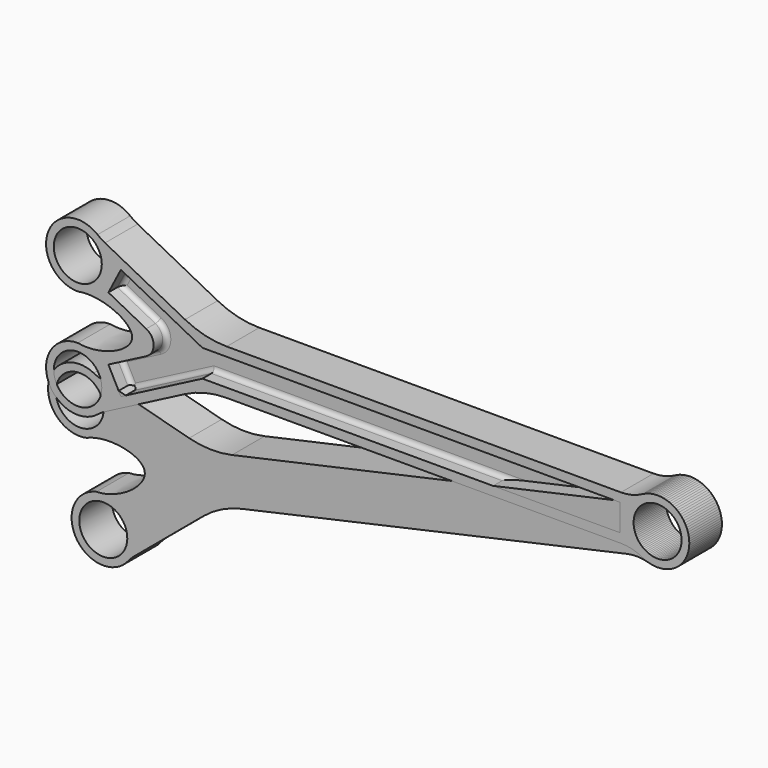
from build123d import *

# Parameters (mm, degrees)
F0_R     = 26.5
F1_DEPTH = 45
F2_ANGLE = 12.5
F4_DEPTH = 17.5
F6_DEPTH = 17.5
F7_R     = 5
F8_R     = 5


with BuildPart() as f1:
    # F0 (on Front) → F1 (new body)
    with BuildSketch(Plane.XZ):
        with BuildLine():
            ThreePointArc((-40.4786778043, -24.7570536722), (-28.191847205, -26.2835209952), (-16.6568059784, -30.7823133406))
            ThreePointArc((-16.6568059784, -30.7823133406), (35, 0), (-16.6568059784, 30.7823133406))
            ThreePointArc((-16.6568059784, 30.7823133406), (-28.191847205, 26.2835209952), (-40.4786778043, 24.7570536722))
            Line((-40.4786778043, 24.7570536722), (-475.6476802408, 24.9871250661))
            ThreePointArc((-475.6476802408, 24.9871250661), (-499.3070169532, 27.8391245956), (-521.6197419488, 36.2081399656))
            Line((-521.6197419488, 36.2081399656), (-609.9031067247, 81.9761380938))
            ThreePointArc((-609.9031067247, 81.9761380938), (-614.1488908448, 84.4491850676), (-618.1314404763, 87.3270215054))
            ThreePointArc((-618.1314404763, 87.3270215054), (-673.0260938705, 71.5878006392), (-640, 25))
            add(Edge.make_bspline(
                [(-640, -25), (-615, -30), (-545, 0), (-615, 30), (-640, 25)],
                knots=[0, 0, 0, 0, 0.5, 1, 1, 1, 1], degree=3))
            ThreePointArc((-640, -25), (-673.0260938705, -71.5878006392), (-618.1314404763, -87.3270215054))
            ThreePointArc((-618.1314404763, -87.3270215054), (-614.1488908449, -84.4491850676), (-609.9031067247, -81.9761380938))
            Line((-609.9031067247, -81.9761380938), (-521.6197419488, -36.2081399656))
            ThreePointArc((-521.6197419488, -36.2081399656), (-499.3070169532, -27.8391245956), (-475.6476802408, -24.9871250661))
            Line((-475.6476802408, -24.9871250661), (-40.4786778043, -24.7570536722))
        make_face()
        with Locations((-640, -60)):
            Circle(F0_R, mode=Mode.SUBTRACT)
        with Locations((-640, 60)):
            Circle(F0_R, mode=Mode.SUBTRACT)
        Circle(F0_R, mode=Mode.SUBTRACT)
    extrude(amount=F1_DEPTH)


with BuildPart() as f2_1:
    # F2: copy of F1
    add(f1.part.rotate(Axis((0, -45, 0), (0, -1, 0)), F2_ANGLE))


with BuildPart() as f1_1:
    add(f1.part)

    # F3 (on face) → F4 (cut)
    with BuildSketch(Plane.XZ.offset(45)):
        with BuildLine():
            Line((-41.5, -14.7575922419), (-41.5, 14.7575922419))
            Line((-41.5, 14.7575922419), (-502.4405189187, 15.001288891))
            Line((-502.4405189187, 15.001288891), (-592.4042612052, 61.6404309199))
            Line((-592.4042612052, 61.6404309199), (-606.2117405459, 35.0067395825))
            Line((-606.2117405459, 35.0067395825), (-564.3734060184, 13.3168456687))
            ThreePointArc((-564.3734060184, 13.3168456687), (-556.2771456888, 0), (-564.3734060184, -13.3168456687))
            Line((-564.3734060184, -13.3168456687), (-606.2117405459, -35.0067395825))
            Line((-606.2117405459, -35.0067395825), (-592.4042612052, -61.6404309199))
            Line((-592.4042612052, -61.6404309199), (-502.4405189187, -15.001288891))
            Line((-502.4405189187, -15.001288891), (-41.5, -14.7575922419))
        make_face()
    extrude(amount=-F4_DEPTH, mode=Mode.SUBTRACT)

    # F5 (on face) → F6 (cut)
    with BuildSketch(Plane(origin=(0, 0, 0), x_dir=(-1, 0, 0), z_dir=(0, 1, 0))):
        with BuildLine():
            Line((502.4405189187, 15.001288891), (41.5, 14.7575922419))
            Line((41.5, 14.7575922419), (41.5, -14.7575922419))
            Line((41.5, -14.7575922419), (502.4405189187, -15.001288891))
            Line((502.4405189187, -15.001288891), (592.4042612052, -61.6404309199))
            Line((592.4042612052, -61.6404309199), (606.2117405459, -35.0067395825))
            Line((606.2117405459, -35.0067395825), (564.3734060184, -13.3168456687))
            ThreePointArc((564.3734060184, -13.3168456687), (556.2771456888, 0), (564.3734060184, 13.3168456687))
            Line((564.3734060184, 13.3168456687), (606.2117405459, 35.0067395825))
            Line((606.2117405459, 35.0067395825), (592.4042612052, 61.6404309199))
            Line((592.4042612052, 61.6404309199), (502.4405189187, 15.001288891))
        make_face()
    extrude(amount=-F6_DEPTH, mode=Mode.SUBTRACT)

    # F7
    f7_edges = [f1_1.edges().sort_by_distance(p)[0] for p in [
        (-271.970259, -17.5, 14.879441),
        (-41.5, -17.5, 0),
        (-271.970259, -17.5, -14.879441),
        (-547.42239, -17.5, 38.32086),
        (-547.42239, -17.5, -38.32086),
        (-599.308001, -17.5, -48.323585),
        (-585.292573, -17.5, -24.161793),
        (-599.308001, -17.5, 48.323585),
    ]]
    fillet(f7_edges, radius=F7_R)

    # F8
    f8_edges = [f1_1.edges().sort_by_distance(p)[0] for p in [
        (-599.308001, -27.5, -48.323585),
        (-547.42239, -27.5, -38.32086),
        (-271.970259, -27.5, -14.879441),
        (-585.292573, -27.5, 24.161793),
        (-599.308001, -27.5, 48.323585),
        (-547.42239, -27.5, 38.32086),
        (-271.970259, -27.5, 14.879441),
        (-41.5, -27.5, 0),
        (-556.277146, -27.5, 0),
        (-585.292573, -27.5, -24.161793),
    ]]
    fillet(f8_edges, radius=F8_R)


with BuildPart() as f9_1:
    # F9: copy of F1
    add(f1_1.part)


solid = Compound([f2_1.part, f1_1.part, f9_1.part])
